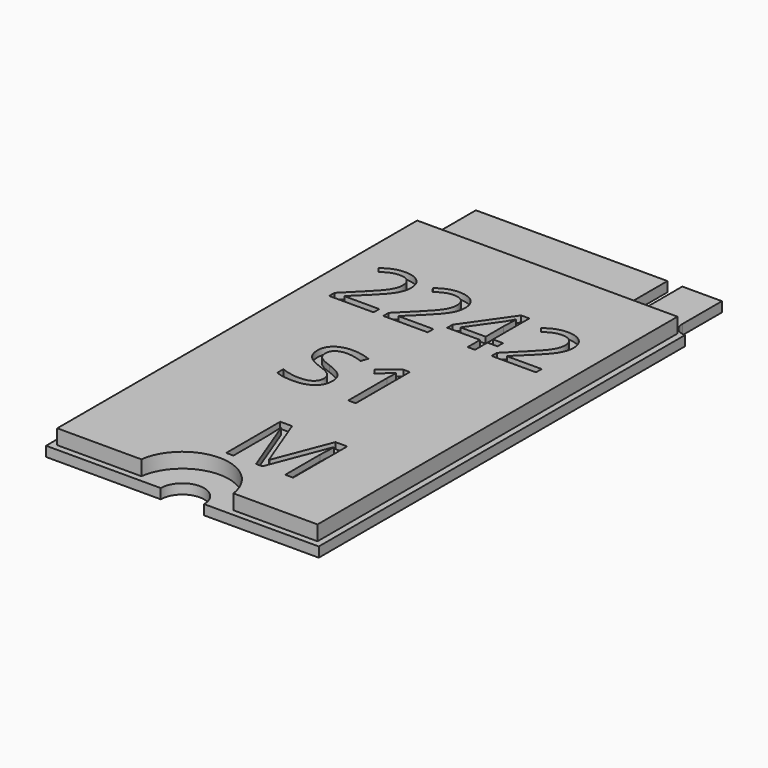
from build123d import *

# Parameters (mm, degrees)
F2_W          = 22
F2_H          = 42
F3_DEPTH      = 0.8
F4_W          = 21
F4_H          = 36.3
F5_DEPTH      = 1.2
F7_DEPTH      = 0.801
F8_R          = 1.75
F9_DEPTH      = 2.001
F11_DEPTH     = 1.2
F12_TEXT_SIZE = 7.6388888889
F13_DEPTH     = 0.5


# Not quite as in the source:
# - Text() gives the source's letters only with a copy of the font that has no kerning and outlines rounded to 1/6400 em; it was checked with that copy


with BuildPart() as f3:
    # F2 (on Top) → F3 (new body)
    with BuildSketch(Plane.XY):
        Rectangle(F2_W, F2_H)
    extrude(amount=F3_DEPTH)

    # F4 (on face) → F5 (join)
    with BuildSketch(Plane.XY.offset(0.8)):
        with Locations((0, -2.35)):
            Rectangle(F4_W, F4_H)
    extrude(amount=F5_DEPTH)

    # F6 (on face) → F7 (cut, through all)
    with BuildSketch(Plane.XY.offset(0.8)):
        with BuildLine():
            Line((-9.925, 17), (-9.925, 21))
            Line((-9.925, 21), (-11, 21))
            Line((-11, 21), (-11, 15.925))
            ThreePointArc((-11, 15.925), (-10.2398602102, 16.2398602102), (-9.925, 17))
        make_face()
        with BuildLine():
            Line((11, 21), (9.925, 21))
            Line((9.925, 21), (9.925, 17))
            ThreePointArc((9.925, 17), (10.2398602102, 16.2398602102), (11, 15.925))
            Line((11, 15.925), (11, 21))
        make_face()
        with BuildLine():
            Line((5.53, 21), (5.53, 17.6))
            ThreePointArc((5.53, 17.6), (6.13, 17), (6.73, 17.6))
            Line((6.73, 17.6), (6.73, 21))
            Line((6.73, 21), (5.53, 21))
        make_face()
    extrude(amount=-F7_DEPTH, mode=Mode.SUBTRACT)

    # F8 (on face) → F9 (cut, through all)
    with BuildSketch(Plane(origin=(0, 0, 0), x_dir=(1, 0, 0), z_dir=(0, 0, -1))):
        with Locations((0, 21)):
            Circle(F8_R)
    extrude(amount=-F9_DEPTH, mode=Mode.SUBTRACT)

    # F10 (on face) → F11 (cut, through all)
    with BuildSketch(Plane.XY.offset(2)):
        with BuildLine():
            ThreePointArc((-1.6770509831, -20.5), (0, -19.25), (1.6770509831, -20.5))
            Line((1.6770509831, -20.5), (3.7165171868, -20.5))
            ThreePointArc((3.7165171868, -20.5), (0, -17.25), (-3.7165171868, -20.5))
            Line((-3.7165171868, -20.5), (-1.6770509831, -20.5))
        make_face()
    extrude(amount=-F11_DEPTH, mode=Mode.SUBTRACT)

    # F12 (on face) → F13 (cut)
    with BuildSketch(Plane.XY.offset(2)):
        with Locations((-8.7775607639, 4.3)):
            Text('2242', F12_TEXT_SIZE, font='Open Sans', text_align=(TextAlign.LEFT, TextAlign.BOTTOM))
        with Locations((-4.8077256944, -6.0888888889)):
            Text('S1', F12_TEXT_SIZE, font='Open Sans', text_align=(TextAlign.LEFT, TextAlign.BOTTOM))
        with Locations((-0.837890625, -16.4777777778)):
            Text('M', F12_TEXT_SIZE, font='Open Sans', text_align=(TextAlign.LEFT, TextAlign.BOTTOM))
    extrude(amount=-F13_DEPTH, mode=Mode.SUBTRACT)


solid = f3.part
